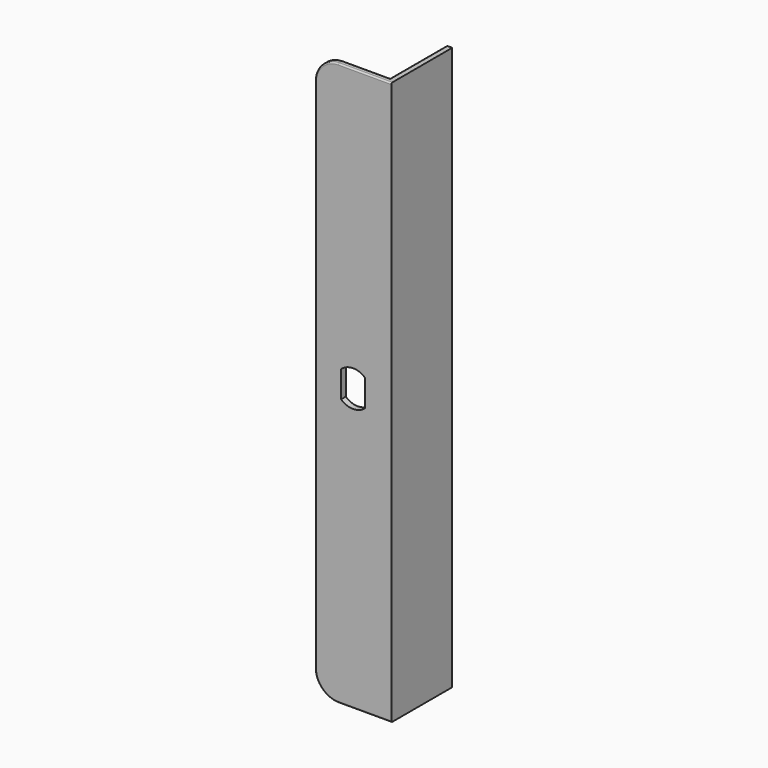
from build123d import *

# Parameters (mm, degrees)
F1_DEPTH     = 304.8
F2_R         = 0.762
F5_DEPTH     = 25.4
F6_R         = 0.381
F7_T1_DEPTH  = 3.175
F7_T4_ANGLE  = 90
F7_T6_ANGLE  = 90
F7_T8_ANGLE  = 90
F7_T10_ANGLE = 90


# Not quite as in the source:
# - a fillet or chamfer that OpenCascade refuses, or shapes differently, is made with other operations: its cross-section is extruded or revolved along the edge and cut away or added


with BuildPart() as f1:
    # F0 (on Top) → F1 (new body)
    with BuildSketch(Plane.XY):
        Polygon((0, 3.175), (0, 0), (41.275, 0), (41.275, 41.275), (38.1, 41.275), (38.1, 3.175), align=None)
    extrude(amount=F1_DEPTH)

    # F2
    f2_edges = [f1.edges().sort_by_distance(p)[0] for p in [
        (0, 0, 152.4),
        (20.6375, 0, 304.8),
        (20.6375, 0, 0),
        (38.1, 22.225, 304.8),
        (19.05, 3.175, 304.8),
        (0, 3.175, 152.4),
        (19.05, 3.175, 0),
        (38.1, 22.225, 0),
        (38.1, 41.275, 152.4),
    ]]
    fillet(f2_edges, radius=F2_R)

    # F4 (on face) → F5 (cut)
    with BuildSketch(Plane.XZ):
        with BuildLine():
            ThreePointArc((27.178, 159.5842048969), (20.6375, 162.1155), (14.097, 159.5842048969))
            Line((14.097, 159.5842048969), (14.097, 145.2157951031))
            ThreePointArc((14.097, 145.2157951031), (20.6375, 142.6845), (27.178, 145.2157951031))
            Line((27.178, 145.2157951031), (27.178, 159.5842048969))
        make_face()
    extrude(amount=-F5_DEPTH, mode=Mode.SUBTRACT)

    # F6
    f6_edges = [f1.edges().sort_by_distance(p)[0] for p in [
        (14.097, 1.5875, 145.215795),
        (14.097, 1.5875, 159.584205),
        (27.178, 1.5875, 159.584205),
        (27.178, 1.5875, 145.215795),
    ]]
    fillet(f6_edges, radius=F6_R)

    # F7: fillet of radius 12.7 on 2 edges, made by hand

    # F7_s2 → F7_t1 (cut)
    with BuildSketch(Plane.XZ.offset(-3.175)):
        with BuildLine():
            ThreePointArc((12.7, 304.8), (3.7197438789, 301.0802561211), (0, 292.1))
            Line((0, 292.1), (0, 304.8))
            Line((0, 304.8), (12.7, 304.8))
        make_face()
        with BuildLine():
            ThreePointArc((12.7, 0), (3.7197438789, 3.7197438789), (0, 12.7))
            Line((0, 12.7), (0, 0))
            Line((0, 0), (12.7, 0))
        make_face()
    extrude(amount=F7_T1_DEPTH, mode=Mode.SUBTRACT)

    # F7_s3 → F7_t4 (revolve, cut)
    with BuildSketch(Plane.YZ.offset(12.7)):
        with BuildLine():
            ThreePointArc((3.175, 0.762), (2.9518153673, 0.2231846327), (2.413, 0))
            Line((2.413, 0), (3.175, 0))
            Line((3.175, 0), (3.175, 0.762))
        make_face()
    revolve(axis=Axis((12.7, 3.175, 12.7), (0, 1, 0)), revolution_arc=F7_T4_ANGLE, mode=Mode.SUBTRACT)

    # F7_s5 → F7_t6 (revolve, cut)
    with BuildSketch(Plane.XY.offset(12.7)):
        with BuildLine():
            ThreePointArc((0.762, 0), (0.2231846327, 0.2231846327), (0, 0.762))
            Line((0, 0.762), (0, 0))
            Line((0, 0), (0.762, 0))
        make_face()
    revolve(axis=Axis((12.7, 0, 12.7), (0, -1, 0)), revolution_arc=F7_T6_ANGLE, mode=Mode.SUBTRACT)

    # F7_s7 → F7_t8 (revolve, cut)
    with BuildSketch(Plane.XY.offset(292.1)):
        with BuildLine():
            ThreePointArc((0.762, 3.175), (0.2231846327, 2.9518153673), (0, 2.413))
            Line((0, 2.413), (0, 3.175))
            Line((0, 3.175), (0.762, 3.175))
        make_face()
    revolve(axis=Axis((12.7, 3.175, 292.1), (0, 1, 0)), revolution_arc=F7_T8_ANGLE, mode=Mode.SUBTRACT)

    # F7_s9 → F7_t10 (revolve, cut)
    with BuildSketch(Plane.YZ.offset(12.7)):
        with BuildLine():
            ThreePointArc((0, 304.038), (0.2231846327, 304.5768153673), (0.762, 304.8))
            Line((0.762, 304.8), (0, 304.8))
            Line((0, 304.8), (0, 304.038))
        make_face()
    revolve(axis=Axis((12.7, 0, 292.1), (0, -1, 0)), revolution_arc=F7_T10_ANGLE, mode=Mode.SUBTRACT)


solid = f1.part
